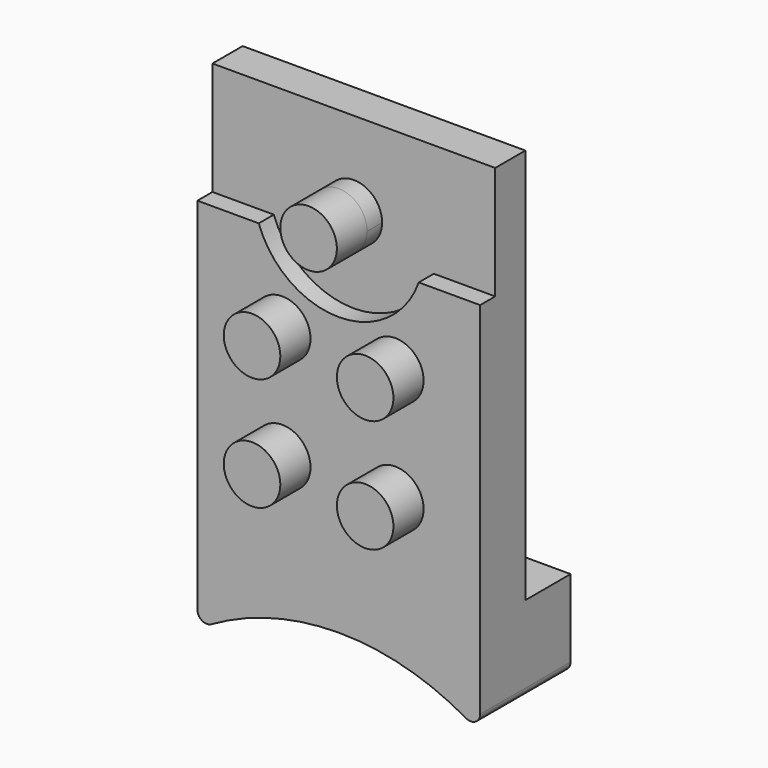
from build123d import *
from build123d import SkipClean  # not in build123d's __all__

# Parameters (mm, degrees)
F0_W      = 15
F0_H      = 15
F0_H_2    = 6
F1_DEPTH  = 10
F2_R      = 1.5
F3_DEPTH  = 2
F5_DEPTH  = 1
F6_R      = 1.5
F7_DEPTH  = 2
F8_W      = 15
F8_H      = 21
F9_DEPTH  = 7
F10_W     = 15
F10_H     = 3
F11_DEPTH = 5
F12_W     = 15
F12_H     = 5
F13_DEPTH = 3
F15_DEPTH = 25
F16_R     = 0.5


# Not quite as in the source:
# - after a boolean that leaves OpenCascade's solid faulty, fix() repairs it


with BuildPart() as f1:
    # F0 (on Front) → F1 (new body)
    with BuildSketch(Plane.XZ):
        Rectangle(F0_W, F0_H)
        with Locations((0, 10.5)):
            Rectangle(F0_W, F0_H_2)
    extrude(amount=F1_DEPTH)

    # F2 (on face) → F3 (join)
    with BuildSketch(Plane.XZ.offset(10)):
        with Locations((-3, 3)):
            Circle(F2_R)
        with Locations((-3, -3)):
            Circle(F2_R)
        with Locations((3, -3)):
            Circle(F2_R)
        with Locations((3, 3)):
            Circle(F2_R)
    extrude(amount=F3_DEPTH)

    # F4 (on face) → F5 (cut)
    with BuildSketch(Plane.XZ.offset(10)):
        with BuildLine():
            Line((-7.5, 13.5), (-7.5, 7.5))
            Line((-7.5, 7.5), (-4.2426406871, 7.5))
            ThreePointArc((-4.2426406871, 7.5), (-3.6742346142, 11.5980762114), (0, 13.5))
            Line((0, 13.5), (-7.5, 13.5))
        make_face()
        with BuildLine():
            ThreePointArc((0, 13.5), (-3.6742346142, 11.5980762114), (-4.2426406871, 7.5))
            Line((-4.2426406871, 7.5), (0, 7.5))
            Line((0, 7.5), (4.2426406871, 7.5))
            ThreePointArc((4.2426406871, 7.5), (4.4351935184, 8.2390410957), (4.5, 9))
            ThreePointArc((4.5, 9), (3.1819805153, 12.1819805153), (0, 13.5))
        make_face()
        with BuildLine():
            ThreePointArc((1.5, 9), (1.0606601718, 7.9393398282), (0, 7.5))
            ThreePointArc((0, 7.5), (-1.0606601718, 10.0606601718), (1.5, 9))
        make_face(mode=Mode.SUBTRACT)
        with BuildLine():
            Line((0, 7.5), (-4.2426406871, 7.5))
            ThreePointArc((-4.2426406871, 7.5), (0, 4.5), (4.2426406871, 7.5))
            Line((4.2426406871, 7.5), (0, 7.5))
        make_face()
        with BuildLine():
            Line((7.5, 13.5), (0, 13.5))
            ThreePointArc((0, 13.5), (3.1819805153, 12.1819805153), (4.5, 9))
            ThreePointArc((4.5, 9), (4.4351935184, 8.2390410957), (4.2426406871, 7.5))
            Line((4.2426406871, 7.5), (7.5, 7.5))
            Line((7.5, 7.5), (7.5, 13.5))
        make_face()
    extrude(amount=-F5_DEPTH, mode=Mode.SUBTRACT)

    # F6 (on face) → F7 (join)
    with BuildSketch(Plane.XZ.offset(10)):
        with Locations((0, 9)):
            Circle(F6_R)
    with SkipClean():  # cleaning this boolean's faces spoils the solid; the shape is the same uncleaned
        extrude(amount=F7_DEPTH)

    # F8 (on face) → F9 (cut)
    with BuildSketch(Plane(origin=(0, 0, 0), x_dir=(-1, 0, 0), z_dir=(0, 1, 0))):
        with Locations((0, 3)):
            Rectangle(F8_W, F8_H)
    extrude(amount=-F9_DEPTH, mode=Mode.SUBTRACT)

    add(f1.part.fix(), mode=Mode.REPLACE)

    # F10 (on face) → F11 (join)
    with BuildSketch(Plane(origin=(0, 0, -7.5), x_dir=(1, 0, 0), z_dir=(0, 0, -1))):
        with Locations((0, 8.5)):
            Rectangle(F10_W, F10_H)
    extrude(amount=F11_DEPTH)

    # F12 (on face) → F13 (join)
    with BuildSketch(Plane(origin=(0, -7, 0), x_dir=(-1, 0, 0), z_dir=(0, 1, 0))):
        with Locations((0, -10)):
            Rectangle(F12_W, F12_H)
    extrude(amount=F13_DEPTH)

    # F14 (on face) → F15 (cut)
    with BuildSketch(Plane(origin=(0, -4, 0), x_dir=(-1, 0, 0), z_dir=(0, 1, 0))):
        with BuildLine():
            Line((-7.5, -12.5), (7.5, -12.5))
            ThreePointArc((7.5, -12.5), (0, -10.237957932), (-7.5, -12.5))
        make_face()
    extrude(amount=-F15_DEPTH, mode=Mode.SUBTRACT)

    # F16
    f16_edges = [f1.edges().sort_by_distance(p)[0] for p in [
        (-7.5, -7, -12.5),
        (7.5, -7, -12.5),
    ]]
    fillet(f16_edges, radius=F16_R)


solid = f1.part
